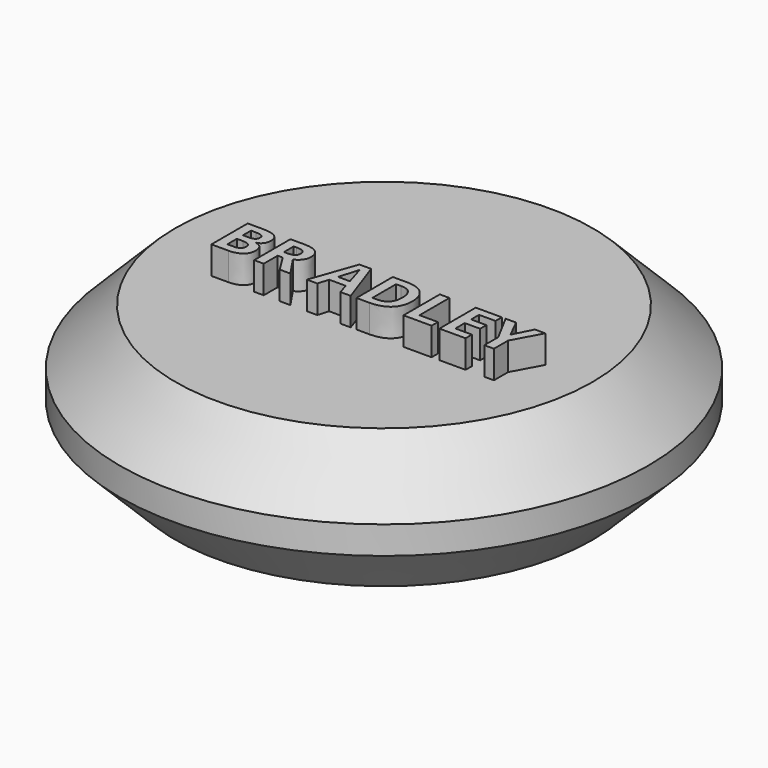
from build123d import *

# Parameters (mm, degrees)
F0_R         = 19
F1_DEPTH     = 10
F2_SIZE      = 4
F3_TEXT_SIZE = 4.5725351898
F4_DEPTH     = 2


# Not quite as in the source:
# - Text() gives the source's letters only with a copy of the font that has no kerning and outlines rounded to 1/6400 em; it was checked with that copy


with BuildPart() as f1:
    # F0 (on Top) → F1 (new body)
    with BuildSketch(Plane.XY):
        Circle(F0_R)
    extrude(amount=F1_DEPTH)

    # F2
    f2_edges = [f1.edges().sort_by_distance(p)[0] for p in [
        (-19, 0, 10),
        (-19, 0, 0),
    ]]
    chamfer(f2_edges, length=F2_SIZE)

    # F3 (on face) → F4 (join)
    with BuildSketch(Plane.XY.offset(10)):
        with Locations((-10.1927295286, -3.2922253366)):
            Text('BR ADLEY', F3_TEXT_SIZE, font='Open Sans', font_style=FontStyle.BOLD, text_align=(TextAlign.LEFT, TextAlign.BOTTOM))
    extrude(amount=F4_DEPTH)


solid = f1.part
